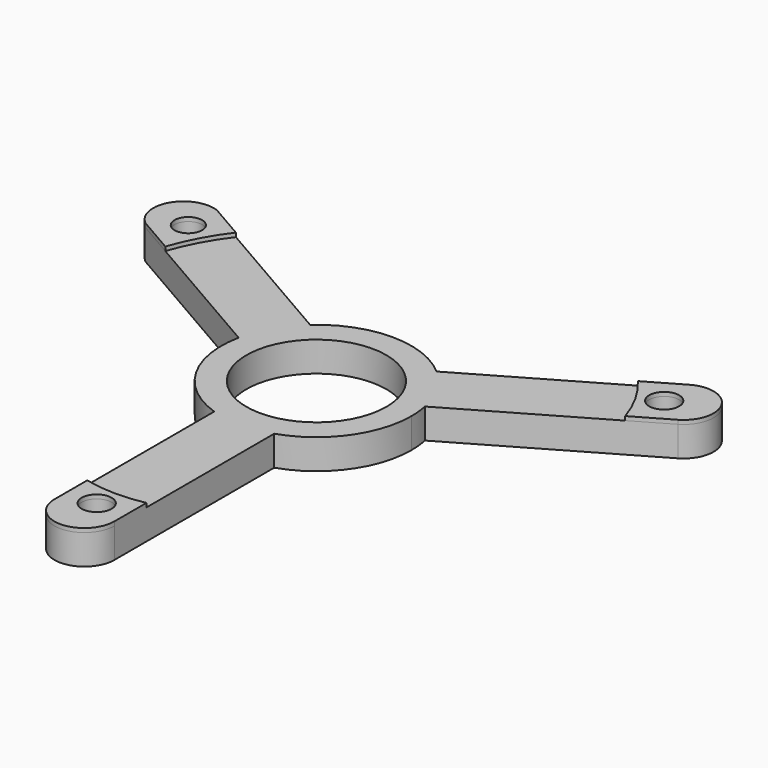
from build123d import *

# Parameters (mm, degrees)
F1_R     = 7.0078592828
F2_DEPTH = 3
F3_R     = 1.3785641614
F3_R_2   = 1.5
F4_DEPTH = 25
F5_R     = 1.3785641614
F5_R_2   = 1.5
F6_DEPTH = 0.4


# Not quite as in the source:
# - a feature names something its author has since deleted; it is built from what else it names


with BuildPart() as f2:
    # F1 (on Top) → F2 (new body)
    with BuildSketch(Plane.XY):
        with BuildLine():
            ThreePointArc((6.3250837122, 7.115890399), (8.2451158332, 4.7603198458), (9.3250837122, 1.9197379763))
            Line((9.3250837122, 1.9197379763), (26.6455917878, 11.9197379763))
            ThreePointArc((26.6455917878, 11.9197379763), (27.7436679992, 16.0178141876), (23.6455917878, 17.115890399))
            Line((23.6455917878, 17.115890399), (6.3250837122, 7.115890399))
        make_face()
        with BuildLine():
            Line((3, -29.0356283753), (3, -9.0356283753))
            ThreePointArc((3, -9.0356283753), (0, -9.5206396916), (-3, -9.0356283753))
            Line((-3, -9.0356283753), (-3, -29.0356283753))
            ThreePointArc((-3, -29.0356283753), (0, -32.0356283753), (3, -29.0356283753))
        make_face()
        with BuildLine():
            ThreePointArc((3, -9.0356283753), (7.7202493228, -5.5713849742), (9.5206396916, 0))
            ThreePointArc((9.5206396916, 0), (9.4716245242, 0.9648362606), (9.3250837122, 1.9197379763))
            ThreePointArc((9.3250837122, 1.9197379763), (8.2451158332, 4.7603198458), (6.3250837122, 7.115890399))
            ThreePointArc((6.3250837122, 7.115890399), (0, 9.5206396916), (-6.3250837122, 7.115890399))
            ThreePointArc((-6.3250837122, 7.115890399), (-8.2451158332, 4.7603198458), (-9.3250837122, 1.9197379763))
            ThreePointArc((-9.3250837122, 1.9197379763), (-8.2451158332, -4.7603198458), (-3, -9.0356283753))
            ThreePointArc((-3, -9.0356283753), (0, -9.5206396916), (3, -9.0356283753))
        make_face()
        Circle(F1_R, mode=Mode.SUBTRACT)
        with BuildLine():
            ThreePointArc((-9.3250837122, 1.9197379763), (-8.2451158332, 4.7603198458), (-6.3250837122, 7.115890399))
            Line((-6.3250837122, 7.115890399), (-23.6455917878, 17.115890399))
            ThreePointArc((-23.6455917878, 17.115890399), (-27.3659550895, 15.7997415376), (-26.6455917878, 11.9197379763))
            Line((-26.6455917878, 11.9197379763), (-9.3250837122, 1.9197379763))
        make_face()
    extrude(amount=F2_DEPTH)

    # F3 (on face) → F4 (cut)
    with BuildSketch(Plane.XY.offset(3)):
        with Locations((-23.8184579752, 13.7452195212)):
            Circle(F3_R)
        with Locations((23.8028700918, 13.7721957361)):
            Circle(F3_R_2)
        with Locations((0, -27.5)):
            Circle(F3_R_2)
    extrude(amount=-F4_DEPTH, mode=Mode.SUBTRACT)

    # F5 (on face) → F6 (join)
    with BuildSketch(Plane.XY.offset(3)):
        with BuildLine():
            ThreePointArc((-22.963211557, 9.7937147588), (-21.7607776153, 12.554595023), (-20.1298891441, 15.0860985312))
            Line((-20.1298891441, 15.0860985312), (-23.6455917878, 17.115890399))
            ThreePointArc((-23.6455917878, 17.115890399), (-27.3659550895, 15.7997415376), (-26.6455917878, 11.9197379763))
            Line((-26.6455917878, 11.9197379763), (-22.963211557, 9.7937147588))
        make_face()
        with Locations((-23.8184579752, 13.7452195212)):
            Circle(F5_R, mode=Mode.SUBTRACT)
        with BuildLine():
            Line((23.6455917878, 17.115890399), (20.1200227065, 15.0804021408))
            ThreePointArc((20.1200227065, 15.0804021408), (21.8423336439, 12.6055758249), (23.0431293377, 9.839855311))
            Line((23.0431293377, 9.839855311), (26.6455917878, 11.9197379763))
            ThreePointArc((26.6455917878, 11.9197379763), (27.7436679992, 16.0178141876), (23.6455917878, 17.115890399))
        make_face()
        with Locations((23.8028700918, 13.7721957361)):
            Circle(F5_R_2, mode=Mode.SUBTRACT)
        with BuildLine():
            ThreePointArc((3, -25.020474568), (-0.0045904533, -25.3057184102), (-3, -24.9363277107))
            Line((-3, -24.9363277107), (-3, -29.0356283753))
            ThreePointArc((-3, -29.0356283753), (0, -32.0356283753), (3, -29.0356283753))
            Line((3, -29.0356283753), (3, -25.020474568))
        make_face()
        with Locations((0, -27.5)):
            Circle(F5_R_2, mode=Mode.SUBTRACT)
    extrude(amount=F6_DEPTH)


solid = f2.part
